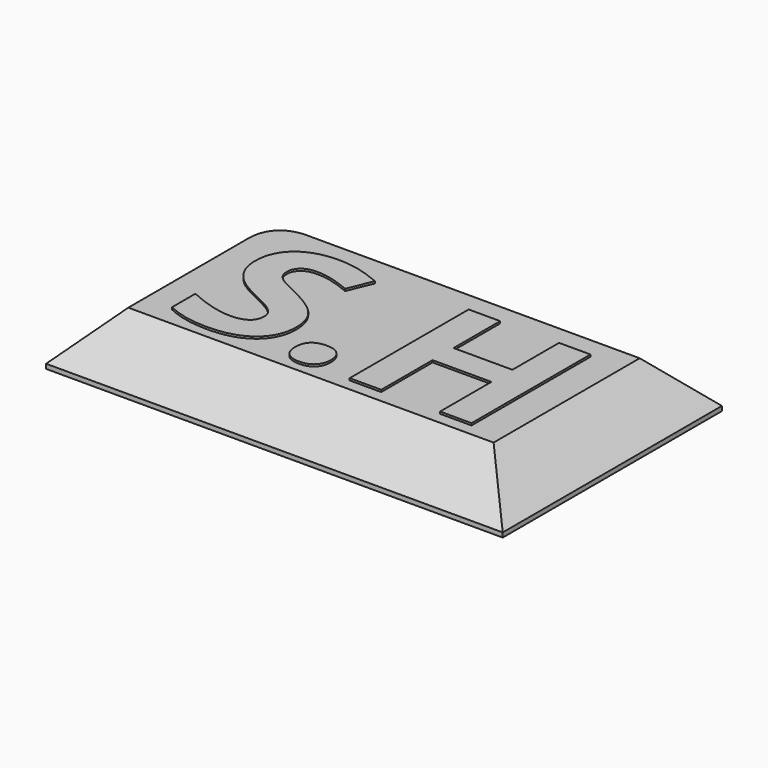
from build123d import *

# Parameters (mm, degrees)
F0_W         = 50.8
F0_H         = 30.48
F1_DEPTH     = 5.588
F2_SIZE      = 5.08
F3_TEXT_SIZE = 23.1697864365
F4_DEPTH     = 5.8166
F5_R         = 1.9606819912
F6_DEPTH     = 25.146
F7_T1_DEPTH  = 17.9966634485
F7_T3_DEPTH  = 15.3353161393


# Not quite as in the source:
# - a fillet or chamfer that OpenCascade refuses, or shapes differently, is made with other operations: its cross-section is extruded or revolved along the edge and cut away or added
# - Text() gives the source's letters only with a copy of the font that has no kerning and outlines rounded to 1/6400 em; it was checked with that copy


with BuildPart() as f1:
    # F0 (on Top) → F1 (new body)
    with BuildSketch(Plane.XY):
        with Locations((25.4, 15.24)):
            Rectangle(F0_W, F0_H)
    extrude(amount=F1_DEPTH)

    # F2
    f2_edges = [f1.edges().sort_by_distance(p)[0] for p in [
        (0, 15.24, 5.588),
        (25.4, 30.48, 5.588),
        (50.8, 15.24, 5.588),
        (25.4, 0, 5.588),
    ]]
    chamfer(f2_edges, length=F2_SIZE)

    # F3 (on Top) → F4 (join)
    with BuildSketch(Plane.XY):
        with Locations((7.2073796764, 6.3975607045)):
            Text('S.H', F3_TEXT_SIZE, font='Open Sans', font_style=FontStyle.BOLD, text_align=(TextAlign.LEFT, TextAlign.BOTTOM))
    extrude(amount=F4_DEPTH)

    # F5 (on Top) → F6 (cut)
    with BuildSketch(Plane.XY):
        with Locations((3.3800282981, 27.2434987128)):
            Circle(F5_R)
    extrude(amount=F6_DEPTH, mode=Mode.SUBTRACT)

    # F7: fillet of radius 5.08 on 2 edges, made by hand

    # F7_s2 → F7_t1 (cut)
    with BuildSketch(Plane(origin=(-14.224, 14.224, -14.224), x_dir=(0.7071067812, 0.7071067812, 0), z_dir=(0.5773502692, -0.5773502692, 0.5773502692))):
        with BuildLine():
            ThreePointArc((19.0126146906, 11.3917184727), (21.5526146906, 12.0723094215), (24.0926146906, 11.3917184727))
            Line((24.0926146906, 11.3917184727), (21.5526146906, 12.8581881564))
            Line((21.5526146906, 12.8581881564), (19.0126146906, 11.3917184727))
        make_face()
    extrude(amount=F7_T1_DEPTH, mode=Mode.SUBTRACT)

    # F7_s4 → F7_t3 (cut)
    with BuildSketch(Plane(origin=(-9.5311822345, 9.5311822345, -9.5311822345), x_dir=(0.7071067812, 0.7071067812, 0), z_dir=(0.5773502692, -0.5773502692, 0.5773502692))):
        with BuildLine():
            ThreePointArc((19.0126146906, 11.3917184727), (21.5526146906, 12.0723094215), (24.0926146906, 11.3917184727))
            Line((24.0926146906, 11.3917184727), (21.5526146906, 12.8581881564))
            Line((21.5526146906, 12.8581881564), (19.0126146906, 11.3917184727))
        make_face()
    extrude(amount=F7_T3_DEPTH, mode=Mode.SUBTRACT)


solid = f1.part
